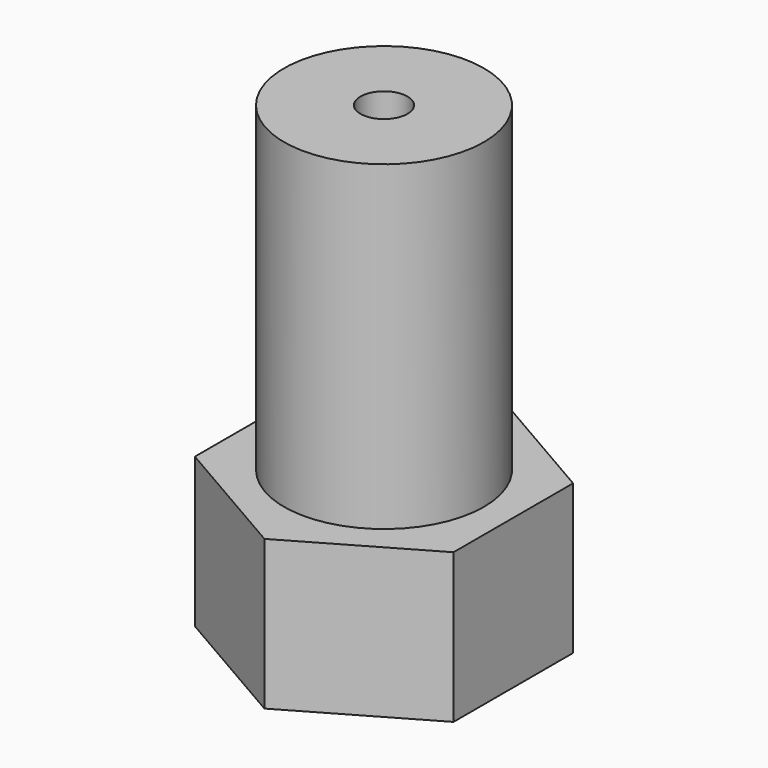
from build123d import *

# Parameters (mm, degrees)
F0_R     = 4.25
F1_DEPTH = 6.35
F0_R_2   = 1
F2_DEPTH = 20


# Not quite as in the source:
# - a feature names something its author has since deleted; it is built from what else it names


with BuildPart() as f1:
    # F0 (on Top) → F1 (new body)
    with BuildSketch(Plane.XY):
        Polygon((5.5011057574, 3.1718053303), (0.0036888868, 6.35), (-5.4974168706, 3.1781946697), (-5.5011057574, -3.1718053303), (-0.0036888868, -6.35), (5.4974168706, -3.1781946697), align=None)
        Circle(F0_R, mode=Mode.SUBTRACT)
    extrude(amount=F1_DEPTH)


with BuildPart() as f2:
    # F0 (on Top) → F2 (new body)
    with BuildSketch(Plane.XY):
        Circle(F0_R)
        Circle(F0_R_2, mode=Mode.SUBTRACT)
    extrude(amount=F2_DEPTH)


solid = Compound([f1.part, f2.part])
